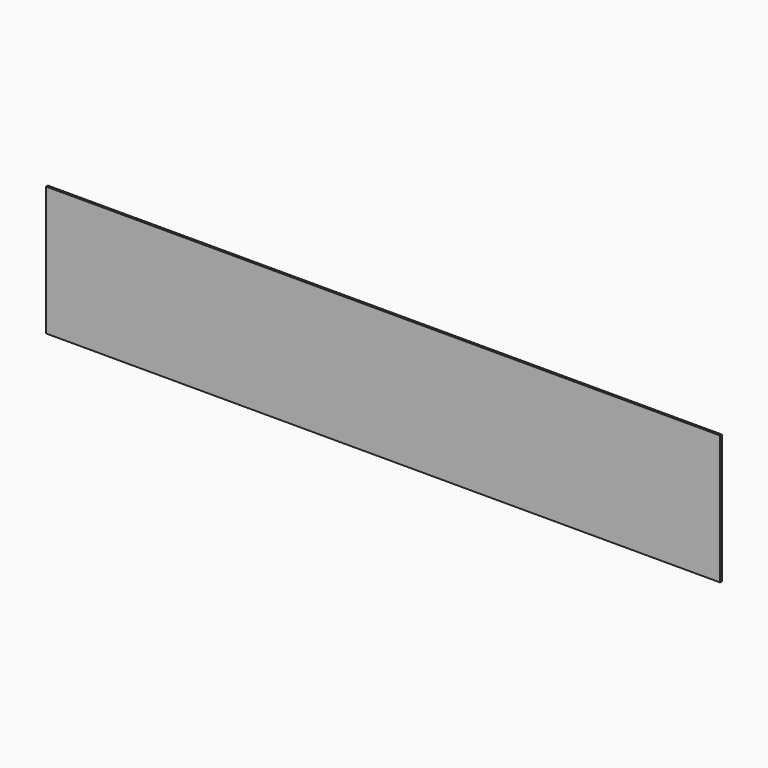
from build123d import *

# Parameters (mm, degrees)
F2_W     = 157.1625
F2_H     = 30.1625
F3_DEPTH = 0.508


# Not quite as in the source:
# - the program builds the solid bodies; features that only make, move or delete a surface that nothing else refers to are left out


with BuildPart() as f3:
    # F2 (on Front) → F3 (new body)
    with BuildSketch(Plane.XZ):
        with Locations((-0.8305758238, 7.4846737444)):
            Rectangle(F2_W, F2_H)
    extrude(amount=F3_DEPTH)


solid = f3.part
